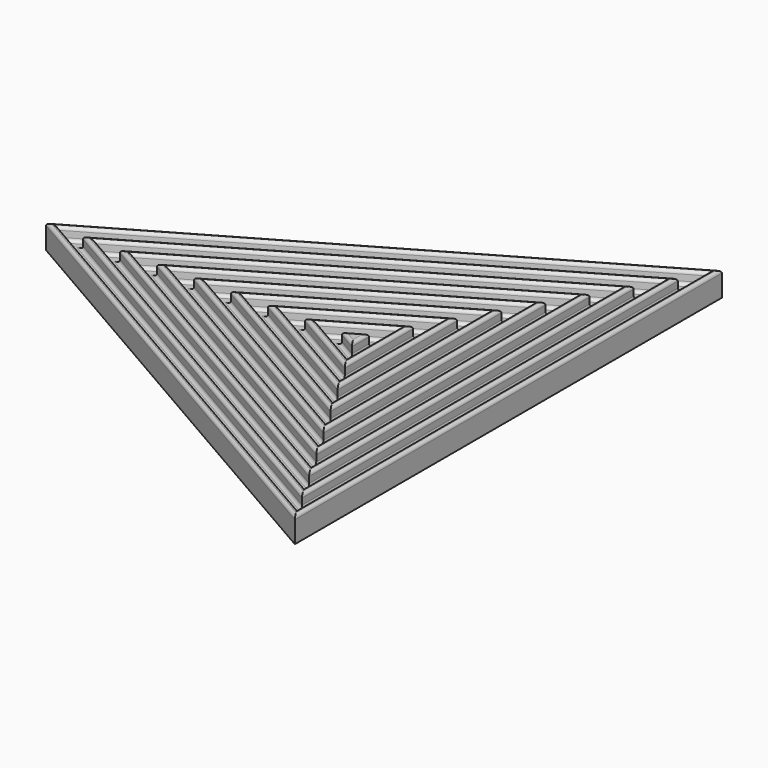
from build123d import *

# Parameters (mm, degrees)
F1_DEPTH = 2.54
F3_DEPTH = 2.54
F4_R     = 0.63499


# Not quite as in the source:
# - a fillet or chamfer is up to 0.001 mm smaller than in the source, because OpenCascade refuses the exact size


with BuildPart() as f1:
    # F0 (on Top) → F1 (new body)
    with BuildSketch(Plane.XY):
        with BuildLine():
            ThreePointArc((-15.8749996872, -27.4963067508), (15.8750001564, -27.4963064799), (31.75, 0))
            ThreePointArc((31.75, 0), (15.8749996133, 27.4963067934), (-15.8750007733, 27.4963061237))
            ThreePointArc((-15.8750007733, 27.4963061237), (-31.75, -6.271e-07), (-15.8749996872, -27.4963067508))
        make_face()
        with BuildLine():
            Line((31.75, -54.9926131403), (31.75, 0))
            ThreePointArc((31.75, 0), (15.8750001564, -27.4963064799), (-15.8749996872, -27.4963067508))
            Line((-15.8749996872, -27.4963067508), (31.75, -54.9926131403))
        make_face()
        with BuildLine():
            ThreePointArc((-15.8750007733, 27.4963061237), (15.8749996133, 27.4963067934), (31.75, 0))
            Line((31.75, 0), (31.75, 54.9926131403))
            Line((31.75, 54.9926131403), (-15.8750007733, 27.4963061237))
        make_face()
        with BuildLine():
            ThreePointArc((-15.8749996872, -27.4963067508), (-31.75, -6.271e-07), (-15.8750007733, 27.4963061237))
            Line((-15.8750007733, 27.4963061237), (-63.5, 0))
            Line((-63.5, 0), (-15.8749996872, -27.4963067508))
        make_face()
    extrude(amount=F1_DEPTH)

    # F2 (on face) → F3 (join)
    with BuildSketch(Plane.XY.offset(2.54)):
        Polygon((31.75, 54.9926131403), (-63.5, 0), (31.75, -54.9926131403), align=None)
        Polygon((30.48, -52.7929086147), (-60.96, 0), (30.48, 52.7929086147), align=None, mode=Mode.SUBTRACT)
        Polygon((27.94, 48.3934995635), (-55.88, 0), (27.94, -48.3934995635), align=None)
        Polygon((-53.34, 0), (26.67, 46.1937950379), (26.67, -46.1937950379), align=None, mode=Mode.SUBTRACT)
        Polygon((24.13, 41.7943859866), (-48.26, 0), (24.13, -41.7943859866), align=None)
        Polygon((22.86, -39.594681461), (-45.72, 0), (22.86, 39.594681461), align=None, mode=Mode.SUBTRACT)
        Polygon((20.32, 35.1952724098), (-40.64, 0), (20.32, -35.1952724098), align=None)
        Polygon((19.05, -32.9955678842), (-38.1, 0), (19.05, 32.9955678842), align=None, mode=Mode.SUBTRACT)
        Polygon((16.51, 28.596158833), (-33.02, 0), (16.51, -28.596158833), align=None)
        Polygon((15.24, -26.3964543073), (-30.48, 0), (15.24, 26.3964543073), align=None, mode=Mode.SUBTRACT)
        Polygon((12.7, 21.9970452561), (-25.4, 0), (12.7, -21.9970452561), align=None)
        Polygon((-22.86, 0), (11.43, 19.7973407305), (11.43, -19.7973407305), align=None, mode=Mode.SUBTRACT)
        Polygon((8.89, -15.3979316793), (8.89, 15.3979316793), (-17.78, 0), align=None)
        Polygon((-15.24, 0), (7.62, 13.1982271537), (7.62, -13.1982271537), align=None, mode=Mode.SUBTRACT)
        Polygon((5.08, -8.7988181024), (5.08, 8.7988181024), (-10.16, 0), align=None)
        Polygon((3.81, -6.5991135768), (-7.62, 0), (3.81, 6.5991135768), align=None, mode=Mode.SUBTRACT)
        Polygon((1.27, 2.1997045256), (-2.54, 0), (1.27, -2.1997045256), align=None)
    extrude(amount=F3_DEPTH)

    # F4 (radius 0.635 in the source; OpenCascade refuses exactly that, so slightly less here)
    f4_edges = [f1.edges().sort_by_distance(p)[0] for p in [
        (-15.875, 27.496307, 5.08),
        (-15.875, -27.496307, 5.08),
        (31.75, 0, 5.08),
        (-15.24, -26.396454, 5.08),
        (-15.24, 26.396454, 5.08),
        (30.48, 0, 5.08),
        (-15.24, -26.396454, 2.54),
        (-15.24, 26.396454, 2.54),
        (30.48, 0, 2.54),
        (27.94, 0, 2.54),
        (-13.97, 24.19675, 2.54),
        (-13.97, -24.19675, 2.54),
        (27.94, 0, 5.08),
        (-13.97, 24.19675, 5.08),
        (-13.97, -24.19675, 5.08),
        (-13.335, -23.096898, 5.08),
        (-13.335, 23.096898, 5.08),
        (26.67, 0, 5.08),
        (-13.335, -23.096898, 2.54),
        (-13.335, 23.096898, 2.54),
        (26.67, 0, 2.54),
        (24.13, 0, 2.54),
        (-12.065, 20.897193, 2.54),
        (-12.065, -20.897193, 2.54),
        (24.13, 0, 5.08),
        (-12.065, 20.897193, 5.08),
        (-12.065, -20.897193, 5.08),
        (-11.43, -19.797341, 5.08),
        (-11.43, 19.797341, 5.08),
        (22.86, 0, 5.08),
        (-11.43, -19.797341, 2.54),
        (-11.43, 19.797341, 2.54),
        (22.86, 0, 2.54),
        (20.32, 0, 2.54),
        (-10.16, 17.597636, 2.54),
        (-10.16, -17.597636, 2.54),
        (20.32, 0, 5.08),
        (-10.16, 17.597636, 5.08),
        (-10.16, -17.597636, 5.08),
        (-9.525, -16.497784, 5.08),
        (-9.525, 16.497784, 5.08),
        (19.05, 0, 5.08),
        (-9.525, -16.497784, 2.54),
        (-9.525, 16.497784, 2.54),
        (19.05, 0, 2.54),
        (-8.255, 14.298079, 2.54),
        (-8.255, -14.298079, 2.54),
        (16.51, 0, 2.54),
        (-8.255, 14.298079, 5.08),
        (-8.255, -14.298079, 5.08),
        (16.51, 0, 5.08),
        (-7.62, -13.198227, 5.08),
        (-7.62, 13.198227, 5.08),
        (15.24, 0, 5.08),
        (-7.62, -13.198227, 2.54),
        (-7.62, 13.198227, 2.54),
        (15.24, 0, 2.54),
        (-6.35, 10.998523, 2.54),
        (-6.35, -10.998523, 2.54),
        (12.7, 0, 2.54),
        (-6.35, 10.998523, 5.08),
        (-6.35, -10.998523, 5.08),
        (12.7, 0, 5.08),
        (-5.715, -9.89867, 5.08),
        (-5.715, 9.89867, 5.08),
        (11.43, 0, 5.08),
        (-5.715, -9.89867, 2.54),
        (-5.715, 9.89867, 2.54),
        (11.43, 0, 2.54),
        (8.89, 0, 2.54),
        (-4.445, 7.698966, 2.54),
        (-4.445, -7.698966, 2.54),
        (8.89, 0, 5.08),
        (-4.445, 7.698966, 5.08),
        (-4.445, -7.698966, 5.08),
        (-3.81, -6.599114, 5.08),
        (-3.81, 6.599114, 5.08),
        (7.62, 0, 5.08),
        (-3.81, -6.599114, 2.54),
        (-3.81, 6.599114, 2.54),
        (7.62, 0, 2.54),
        (5.08, 0, 2.54),
        (-2.54, 4.399409, 2.54),
        (-2.54, -4.399409, 2.54),
        (5.08, 0, 5.08),
        (-2.54, 4.399409, 5.08),
        (-2.54, -4.399409, 5.08),
        (-1.905, -3.299557, 5.08),
        (-1.905, 3.299557, 5.08),
        (3.81, 0, 5.08),
        (-1.905, -3.299557, 2.54),
        (-1.905, 3.299557, 2.54),
        (3.81, 0, 2.54),
        (1.27, 0, 2.54),
        (-0.635, 1.099852, 2.54),
        (-0.635, -1.099852, 2.54),
        (1.27, 0, 5.08),
        (-0.635, 1.099852, 5.08),
        (-0.635, -1.099852, 5.08),
    ]]
    fillet(f4_edges, radius=F4_R)


solid = f1.part
